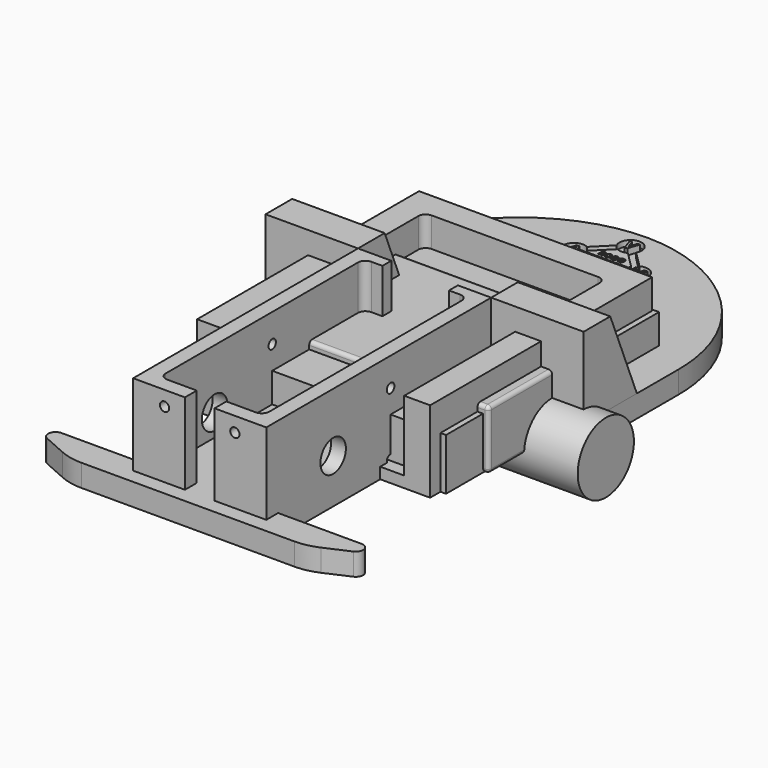
from build123d import *

# Parameters (mm, degrees)
F0_W          = 69
F0_H          = 43
F1_DEPTH      = 16
F2_R          = 1
F3_R          = 9.5
F4_DEPTH      = 49
F6_DEPTH      = 14
F8_DEPTH      = 6
F9_W          = 5
F9_H          = 3
F10_DEPTH     = 22
F11_W         = 14
F11_H         = 22
F12_DEPTH     = 4
F13_W         = 63
F13_H         = 75
F14_DEPTH     = 3
F15_W         = 49
F15_H         = 7
F16_DEPTH     = 19
F18_DEPTH     = 25
F20_DEPTH     = 25
F21_R         = 1.25
F21_R_2       = 4.325169796
F22_DEPTH     = 10
F23_R         = 4.3011723368
F23_R_2       = 1.2554899624
F23_R_3       = 1.2772053527
F24_DEPTH     = 10
F25_R         = 1.25
F26_DEPTH     = 5
F27_R         = 2
F28_R         = 2
F29_TEXT_SIZE = 2.3611111111
F30_DEPTH     = 1.5
F31_TEXT_SIZE = 4.1666666667
F32_DEPTH     = 1.7


# Not quite as in the source:
# - Text() gives the source's letters only with a copy of the font that has no kerning and outlines rounded to 1/6400 em; it was checked with that copy


with BuildPart() as f1:
    # F0 (on Top) → F1 (new body)
    with BuildSketch(Plane.XY):
        Rectangle(F0_W, F0_H)
    extrude(amount=F1_DEPTH)

    # F2
    f2_edges = [f1.edges().sort_by_distance(p)[0] for p in [
        (-34.5, 21.5, 8),
        (34.5, -21.5, 8),
        (-34.5, -21.5, 8),
        (0, -21.5, 0),
        (34.5, 0, 16),
        (-34.5, 0, 0),
        (-34.5, 0, 16),
        (34.5, 21.5, 8),
        (0, 21.5, 0),
        (0, 21.5, 16),
        (0, -21.5, 16),
        (34.5, 0, 0),
    ]]
    fillet(f2_edges, radius=F2_R)


with BuildPart() as f4:
    # F3 (on Right) → F4 (new body)
    with BuildSketch(Plane.YZ):
        Circle(F3_R)
    extrude(amount=F4_DEPTH)


with BuildPart() as f6:
    # F5 (on Top) → F6 (new body)
    with BuildSketch(Plane.XY):
        Polygon((33, -34), (33, 38), (26, 38), (25, 39), (-12, 39), (-14.1213203436, 36.8786796564), (-27.1213203436, 36.8786796564), (-30, 34), (-30, -34), align=None)
    extrude(amount=F6_DEPTH)


with BuildPart() as f8:
    # F7 (on Top) → F8 (new body)
    with BuildSketch(Plane.XY):
        with BuildLine():
            Line((-18, 0), (-18, -72))
            Line((-18, -72), (-40.5755710991, -72))
            ThreePointArc((-40.5755710991, -72), (-42.5320023136, -73.584817025), (-41.3878480312, -75.8276230972))
            Line((-41.3878480312, -75.8276230972), (-34.9088602341, -78.7071732293))
            ThreePointArc((-34.9088602341, -78.7071732293), (-31.930655556, -79.6732341091), (-28.8167832433, -80))
            Line((-28.8167832433, -80), (0, -80))
            Line((0, -80), (28.8167832433, -80))
            ThreePointArc((28.8167832433, -80), (31.930655556, -79.6732341091), (34.9088602341, -78.7071732293))
            Line((34.9088602341, -78.7071732293), (41.3878480312, -75.8276230972))
            ThreePointArc((41.3878480312, -75.8276230972), (42.5320023136, -73.584817025), (40.5755710991, -72))
            Line((40.5755710991, -72), (18, -72))
            Line((18, -72), (18, 0))
            Line((18, 0), (43, 0))
            Line((43, 0), (43, 32))
            add(Edge.make_bspline(
                [(-43, 32), (-43, 57), (0, 93), (43, 57), (43, 32)],
                knots=[0, 0, 0, 0, 0.5, 1, 1, 1, 1], degree=3))
            Line((-43, 32), (-43, 0))
            Line((-43, 0), (-18, 0))
        make_face()
    extrude(amount=F8_DEPTH)

    # F9 (on face) → F10 (join)
    with BuildSketch(Plane.XY.offset(6)):
        Polygon((18, -72), (18, 0), (14, 0), (14, -3), (14, -72), align=None)
        with Locations((11.5, -1.5)):
            Rectangle(F9_W, F9_H)
        Polygon((-14, 0), (-18, 0), (-18, -72), (-14, -72), (-14, -3), align=None)
        with Locations((-11.5, -1.5)):
            Rectangle(F9_W, F9_H)
    extrude(amount=F10_DEPTH)

    # F11 (on face) → F12 (join)
    with BuildSketch(Plane.XZ.offset(72)):
        with Locations((11, 17)):
            Rectangle(F11_W, F11_H)
        with Locations((-11, 17)):
            Rectangle(F11_W, F11_H)
    extrude(amount=F12_DEPTH)

    # F21 (on face) → F22 (cut)
    with BuildSketch(Plane(origin=(-18, 0, 0), x_dir=(0, -1, 0), z_dir=(-1, 0, 0))):
        with Locations((33.9965857565, 20.3136056662)):
            Circle(F21_R)
        with BuildLine():
            ThreePointArc((34.0027213097, 2.0456765499), (34.8866047861, 2.4117930734), (35.2527213097, 3.2956765499))
            ThreePointArc((35.2527213097, 3.2956765499), (33.1188378332, 4.1795600264), (34.0027213097, 2.0456765499))
        make_face()
        with Locations((53.4486211836, 12)):
            Circle(F21_R_2)
    extrude(amount=-F22_DEPTH, mode=Mode.SUBTRACT)

    # F23 (on face) → F24 (cut)
    with BuildSketch(Plane.YZ.offset(18)):
        with Locations((-53.4013621509, 12.0410323143)):
            Circle(F23_R)
        with Locations((-34.0310148895, 3.3050463535)):
            Circle(F23_R_2)
        with Locations((-33.9883118868, 20.287271589)):
            Circle(F23_R_3)
    extrude(amount=-F24_DEPTH, mode=Mode.SUBTRACT)

    # F25 (on face) → F26 (cut)
    with BuildSketch(Plane.XZ.offset(76)):
        with Locations((-9.5, 24)):
            Circle(F25_R)
        with Locations((9.5, 24)):
            Circle(F25_R)
    extrude(amount=-F26_DEPTH, mode=Mode.SUBTRACT)

    # F27
    f27_edges = [f8.edges().sort_by_distance(p)[0] for p in [
        (-14, -72, 17),
        (14, -72, 17),
        (-14, -3, 17),
        (14, -3, 17),
    ]]
    fillet(f27_edges, radius=F27_R)

    # F29 (on face) → F30 (cut)
    with BuildSketch(Plane.XY.offset(6)):
        with BuildLine():
            ThreePointArc((2.6499255667, 68.2041224768), (2.9111661495, 68.8858529666), (3, 69.6104988456))
            ThreePointArc((3, 69.6104988456), (-0.724645879, 72.5216649951), (-2.6499255667, 68.2041224768))
            Line((-2.6499255667, 68.2041224768), (-1.2647186258, 69.5893294177))
            Line((-1.2647186258, 69.5893294177), (-1.2352813742, 69.5893294177))
            Line((-1.2352813742, 69.5893294177), (1.2352813742, 69.5893294177))
            Line((1.2352813742, 69.5893294177), (1.2647186258, 69.5893294177))
            Line((1.2647186258, 69.5893294177), (2.6499255667, 68.2041224768))
        make_face()
        with BuildLine():
            Line((-1.2647186258, 69.5893294177), (-2.6499255667, 68.2041224768))
            ThreePointArc((-2.6499255667, 68.2041224768), (-2.117942438, 67.4858059667), (-1.3979366965, 66.956111347))
            Line((-1.3979366965, 66.956111347), (0, 68.3540480435))
            Line((0, 68.3540480435), (-1.2352813742, 69.5893294177))
            Line((-1.2352813742, 69.5893294177), (-1.2647186258, 69.5893294177))
        make_face()
        with BuildLine():
            ThreePointArc((-1.3979366965, 66.956111347), (-2.117942438, 67.4858059667), (-2.6499255667, 68.2041224768))
            Line((-2.6499255667, 68.2041224768), (-7.0978406575, 63.756207386))
            ThreePointArc((-7.0978406575, 63.756207386), (-6.3786796564, 63.225368387), (-5.8478406575, 62.506207386))
            Line((-5.8478406575, 62.506207386), (-1.3979366965, 66.956111347))
        make_face()
        with BuildLine():
            Line((7.0978406575, 63.756207386), (2.6499255667, 68.2041224768))
            ThreePointArc((2.6499255667, 68.2041224768), (2.117942438, 67.4858059667), (1.3979366965, 66.956111347))
            Line((1.3979366965, 66.956111347), (5.8478406575, 62.506207386))
            ThreePointArc((5.8478406575, 62.506207386), (6.3786796564, 63.225368387), (7.0978406575, 63.756207386))
        make_face()
        with BuildLine():
            ThreePointArc((1.3979366965, 66.956111347), (2.117942438, 67.4858059667), (2.6499255667, 68.2041224768))
            Line((2.6499255667, 68.2041224768), (1.2647186258, 69.5893294177))
            Line((1.2647186258, 69.5893294177), (1.2352813742, 69.5893294177))
            Line((1.2352813742, 69.5893294177), (0, 68.3540480435))
            Line((0, 68.3540480435), (1.3979366965, 66.956111347))
        make_face()
        with BuildLine():
            Line((-9.75, 61.1040480435), (-7.0978406575, 63.756207386))
            ThreePointArc((-7.0978406575, 63.756207386), (-11.2435164493, 59.8903275269), (-5.5943340588, 60.3576530822))
            Line((-5.5943340588, 60.3576530822), (-8.5, 60.3576530822))
            Line((-8.5, 60.3576530822), (-8.5, 61.1040480435))
            Line((-8.5, 61.1040480435), (-9.75, 61.1040480435))
        make_face()
        with BuildLine():
            ThreePointArc((-5.8478406575, 62.506207386), (-6.3786796564, 63.225368387), (-7.0978406575, 63.756207386))
            Line((-7.0978406575, 63.756207386), (-9.75, 61.1040480435))
            Line((-9.75, 61.1040480435), (-8.5, 61.1040480435))
            Line((-8.5, 61.1040480435), (-8.5, 61.8504430047))
            Line((-8.5, 61.8504430047), (-6.5036050388, 61.8504430047))
            Line((-6.5036050388, 61.8504430047), (-5.8478406575, 62.506207386))
        make_face()
        with BuildLine():
            Line((9.75, 61.1040480435), (7.0978406575, 63.756207386))
            ThreePointArc((7.0978406575, 63.756207386), (6.3786796564, 63.225368387), (5.8478406575, 62.506207386))
            Line((5.8478406575, 62.506207386), (6.5036050388, 61.8504430047))
            Line((6.5036050388, 61.8504430047), (8.5, 61.8504430047))
            Line((8.5, 61.8504430047), (8.5, 61.1040480435))
            Line((8.5, 61.1040480435), (9.75, 61.1040480435))
        make_face()
        with BuildLine():
            ThreePointArc((11.5, 61.1040480435), (10.0481475983, 63.6737248741), (7.0978406575, 63.756207386))
            Line((7.0978406575, 63.756207386), (9.75, 61.1040480435))
            Line((9.75, 61.1040480435), (8.5, 61.1040480435))
            Line((8.5, 61.1040480435), (8.5, 60.3576530822))
            Line((8.5, 60.3576530822), (5.5943340588, 60.3576530822))
            ThreePointArc((5.5943340588, 60.3576530822), (8.8761663039, 58.1277249912), (11.5, 61.1040480435))
        make_face()
        with BuildLine():
            Line((-8.5, 60.3576530822), (-5.5943340588, 60.3576530822))
            ThreePointArc((-5.5943340588, 60.3576530822), (-5.5236769477, 60.7278817396), (-5.5, 61.1040480435))
            ThreePointArc((-5.5, 61.1040480435), (-5.5236769477, 61.4802143474), (-5.5943340588, 61.8504430047))
            Line((-5.5943340588, 61.8504430047), (-6.5036050388, 61.8504430047))
            Line((-6.5036050388, 61.8504430047), (-7.25, 61.1040480435))
            Line((-7.25, 61.1040480435), (-8.5, 61.1040480435))
            Line((-8.5, 61.1040480435), (-8.5, 60.3576530822))
        make_face()
        with BuildLine():
            ThreePointArc((-5.5, 61.1040480435), (-5.5236769477, 60.7278817396), (-5.5943340588, 60.3576530822))
            Line((-5.5943340588, 60.3576530822), (5.5943340588, 60.3576530822))
            ThreePointArc((5.5943340588, 60.3576530822), (5.5, 61.1040480435), (5.5943340588, 61.8504430047))
            Line((5.5943340588, 61.8504430047), (-5.5943340588, 61.8504430047))
            ThreePointArc((-5.5943340588, 61.8504430047), (-5.5236769477, 61.4802143474), (-5.5, 61.1040480435))
        make_face()
        with BuildLine():
            ThreePointArc((5.5943340588, 61.8504430047), (5.5, 61.1040480435), (5.5943340588, 60.3576530822))
            Line((5.5943340588, 60.3576530822), (8.5, 60.3576530822))
            Line((8.5, 60.3576530822), (8.5, 61.1040480435))
            Line((8.5, 61.1040480435), (7.25, 61.1040480435))
            Line((7.25, 61.1040480435), (6.5036050388, 61.8504430047))
            Line((6.5036050388, 61.8504430047), (5.5943340588, 61.8504430047))
        make_face()
        Polygon((-1.2352813742, 69.5893294177), (0, 68.3540480435), (1.2352813742, 69.5893294177), align=None)
        with BuildLine():
            Line((0, 68.3540480435), (-1.3979366965, 66.956111347))
            ThreePointArc((-1.3979366965, 66.956111347), (0, 66.6104988456), (1.3979366965, 66.956111347))
            Line((1.3979366965, 66.956111347), (0, 68.3540480435))
        make_face()
        Polygon((-7.25, 61.1040480435), (-6.5036050388, 61.8504430047), (-8.5, 61.8504430047), (-8.5, 61.1040480435), align=None)
        Polygon((8.5, 61.8504430047), (6.5036050388, 61.8504430047), (7.25, 61.1040480435), (8.5, 61.1040480435), align=None)
        with BuildLine():
            ThreePointArc((-5.5943340588, 61.8504430047), (-5.7018109067, 62.1857771214), (-5.8478406575, 62.506207386))
            Line((-5.8478406575, 62.506207386), (-6.5036050388, 61.8504430047))
            Line((-6.5036050388, 61.8504430047), (-5.5943340588, 61.8504430047))
        make_face()
        with Locations((-3.4949070051, 62.6089637162)):
            Text('ROBO', F29_TEXT_SIZE, font='Open Sans', font_style=FontStyle.BOLD, text_align=(TextAlign.LEFT, TextAlign.BOTTOM))
        with BuildLine():
            Line((6.5036050388, 61.8504430047), (5.8478406575, 62.506207386))
            ThreePointArc((5.8478406575, 62.506207386), (5.7018109067, 62.1857771214), (5.5943340588, 61.8504430047))
            Line((5.5943340588, 61.8504430047), (6.5036050388, 61.8504430047))
        make_face()
    extrude(amount=-F30_DEPTH, mode=Mode.SUBTRACT)

    # F31 (on face) → F32 (join)
    with BuildSketch(Plane.XY.offset(4.5)):
        with Locations((-1.4889322917, 68.2482980993)):
            Text('V', F31_TEXT_SIZE, font='Open Sans', font_style=FontStyle.BOLD, text_align=(TextAlign.LEFT, TextAlign.BOTTOM))
        with Locations((-10.0530986669, 59.7122805542)):
            Text('A', F31_TEXT_SIZE, font='Open Sans', font_style=FontStyle.BOLD, text_align=(TextAlign.LEFT, TextAlign.BOTTOM))
        with Locations((6.6133312133, 59.6801674822)):
            Text('M', F31_TEXT_SIZE, font='Open Sans', font_style=FontStyle.BOLD, text_align=(TextAlign.LEFT, TextAlign.BOTTOM))
    extrude(amount=F32_DEPTH)


with BuildPart() as f14:
    # F13 (on Top) → F14 (new body)
    with BuildSketch(Plane.XY):
        Rectangle(F13_W, F13_H)
    extrude(amount=F14_DEPTH)

    # F15 (on face) → F16 (join)
    with BuildSketch(Plane.XY.offset(3)):
        Polygon((-24.5, 37.5), (-31.5, 37.5), (-31.5, -37.5), (-24.5, -37.5), (-24.5, 30.5), align=None)
        Polygon((31.5, 37.5), (24.5, 37.5), (24.5, 30.5), (24.5, -37.5), (31.5, -37.5), align=None)
        with Locations((0, 34)):
            Rectangle(F15_W, F15_H)
    extrude(amount=F16_DEPTH)

    # F28
    f28_edges = [f14.edges().sort_by_distance(p)[0] for p in [
        (-24.5, 30.5, 12.5),
        (24.5, 30.5, 12.5),
    ]]
    fillet(f28_edges, radius=F28_R)


with BuildPart() as f18:
    # F17 (on face) → F18 (new body)
    with BuildSketch(Plane(origin=(-18, 0, 0), x_dir=(0, -1, 0), z_dir=(-1, 0, 0))):
        Polygon((-18, 6), (0, 6), (0, 28), (-9, 28), align=None)
    extrude(amount=F18_DEPTH)


with BuildPart() as f20:
    # F19 (on face) → F20 (new body)
    with BuildSketch(Plane.YZ.offset(18)):
        Polygon((9, 28), (0, 28), (0, 6), (18, 6), align=None)
    extrude(amount=F20_DEPTH)


solid = Compound([f1.part, f4.part, f6.part, f8.part, f14.part, f18.part, f20.part])
